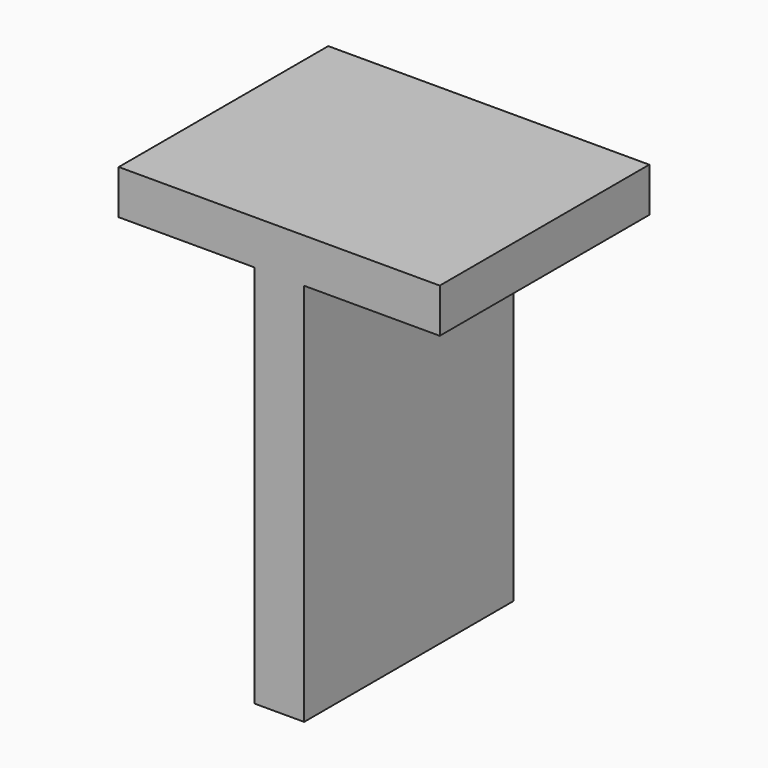
from build123d import *

# Parameters (mm, degrees)
F0_TEXT_SIZE = 58.1793538812
F1_DEPTH     = 25.4


# Not quite as in the source:
# - Text() gives the source's letters only with a copy of the font that has no kerning and outlines rounded to 1/6400 em; it was checked with that copy


with BuildPart() as f1:
    # F0 (on Front) → F1 (new body)
    with BuildSketch(Plane.XZ):
        with Locations((-39.21110183, 0)):
            Text('T', F0_TEXT_SIZE, font='Open Sans', text_align=(TextAlign.LEFT, TextAlign.BOTTOM))
    extrude(amount=F1_DEPTH)


solid = f1.part
